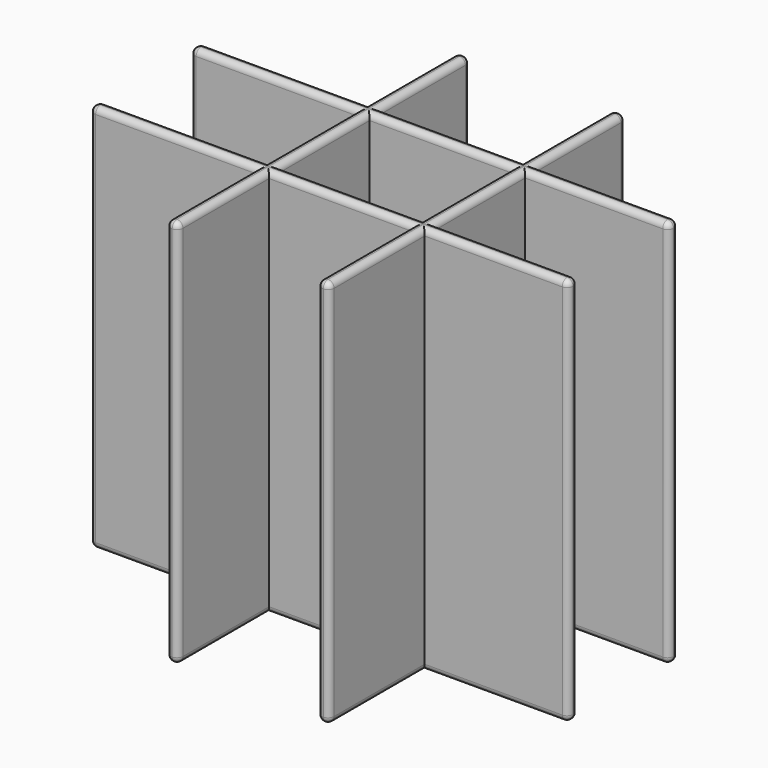
from build123d import *

# Parameters (mm, degrees)
F0_W     = 2
F0_H     = 19
F0_W_2   = 28
F0_H_2   = 2
F0_W_3   = 24
F0_H_3   = 19.9385005981
F1_DEPTH = 65
F2_R     = 0.99999


# Not quite as in the source:
# - a fillet or chamfer is up to 0.001 mm smaller than in the source, because OpenCascade refuses the exact size


with BuildPart() as f1:
    # F0 (on Top) → F1 (new body)
    with BuildSketch(Plane.XY):
        with Locations((29, 32.5)):
            Rectangle(F0_W, F0_H)
        with Locations((14, 22)):
            Rectangle(F0_W_2, F0_H_2)
        with Locations((42, 22)):
            Rectangle(F0_W_3, F0_H_2)
        with Locations((55, 32.5)):
            Rectangle(F0_W, F0_H)
        with Locations((55, 22)):
            Rectangle(F0_W, F0_H_2)
        with Locations((68, 22)):
            Rectangle(F0_W_3, F0_H_2)
        with Locations((68, 1)):
            Rectangle(F0_W_3, F0_H_2)
        with Locations((55, 1)):
            Rectangle(F0_W, F0_H_2)
        with Locations((42, 1)):
            Rectangle(F0_W_3, F0_H_2)
        with Locations((14, 1)):
            Rectangle(F0_W_2, F0_H_2)
        with Locations((29, 1)):
            Rectangle(F0_W, F0_H_2)
        with Locations((29, 11.5)):
            Rectangle(F0_W, F0_H)
        with Locations((29, -9.5)):
            Rectangle(F0_W, F0_H)
        with Locations((55, -9.969250299)):
            Rectangle(F0_W, F0_H_3)
        with Locations((29, 22)):
            Rectangle(F0_W, F0_H_2)
        with Locations((55, 11.5)):
            Rectangle(F0_W, F0_H)
    extrude(amount=F1_DEPTH)

    # F2 (radius 1 in the source; OpenCascade refuses exactly that, so slightly less here)
    f2_edges = [f1.edges().sort_by_distance(p)[0] for p in [
        (28, 32.5, 65),
        (14, 23, 65),
        (0, 22, 65),
        (14, 21, 65),
        (28, 11.5, 65),
        (14, 2, 65),
        (0, 1, 65),
        (14, 0, 65),
        (28, -9.5, 65),
        (29, -19, 65),
        (30, -9.5, 65),
        (42, 0, 65),
        (54, -9.96925, 65),
        (55, -19.938501, 65),
        (56, -9.96925, 65),
        (68, 0, 65),
        (80, 1, 65),
        (68, 2, 65),
        (56, 11.5, 65),
        (68, 21, 65),
        (80, 22, 65),
        (68, 23, 65),
        (56, 32.5, 65),
        (55, 42, 65),
        (54, 32.5, 65),
        (42, 23, 65),
        (30, 32.5, 65),
        (29, 42, 65),
        (42, 2, 65),
        (30, 11.5, 65),
        (42, 21, 65),
        (54, 11.5, 65),
        (28, 32.5, 0),
        (14, 23, 0),
        (0, 22, 0),
        (14, 21, 0),
        (28, 11.5, 0),
        (14, 2, 0),
        (0, 1, 0),
        (14, 0, 0),
        (28, -9.5, 0),
        (29, -19, 0),
        (30, -9.5, 0),
        (42, 0, 0),
        (54, -9.96925, 0),
        (55, -19.938501, 0),
        (56, -9.96925, 0),
        (68, 0, 0),
        (80, 1, 0),
        (68, 2, 0),
        (56, 11.5, 0),
        (68, 21, 0),
        (80, 22, 0),
        (68, 23, 0),
        (56, 32.5, 0),
        (55, 42, 0),
        (54, 32.5, 0),
        (42, 23, 0),
        (30, 32.5, 0),
        (29, 42, 0),
        (42, 2, 0),
        (30, 11.5, 0),
        (42, 21, 0),
        (54, 11.5, 0),
        (30, 42, 32.5),
        (28, 42, 32.5),
        (56, 42, 32.5),
        (54, 42, 32.5),
        (0, 23, 32.5),
        (0, 21, 32.5),
        (0, 2, 32.5),
        (0, 0, 32.5),
        (28, -19, 32.5),
        (30, -19, 32.5),
        (54, -19.938501, 32.5),
        (56, -19.938501, 32.5),
        (80, 0, 32.5),
        (80, 2, 32.5),
        (80, 21, 32.5),
        (80, 23, 32.5),
    ]]
    fillet(f2_edges, radius=F2_R)


solid = f1.part
